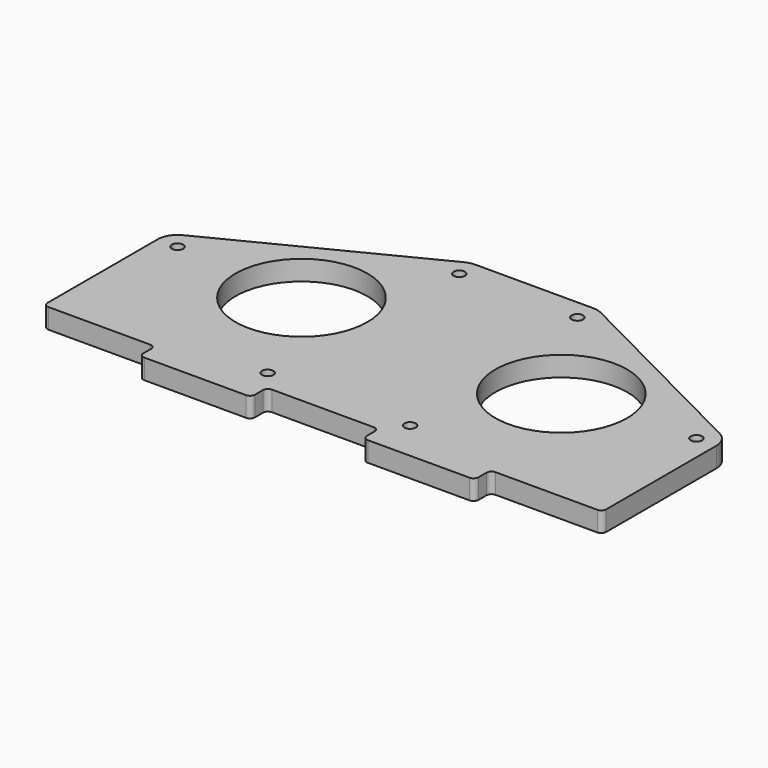
from build123d import *

# Parameters (mm, degrees)
F0_R     = 3.6195
F0_R_2   = 41.94175
F1_DEPTH = 12.7
F2_W     = 71.12
F2_H     = 12.7
F3_DEPTH = 12.7
F4_R     = 3.175


with BuildPart() as f1:
    # F0 (on Top) → F1 (new body)
    with BuildSketch(Plane.XY):
        with BuildLine():
            Line((37.5943482574, 0), (-37.5943482574, 0))
            ThreePointArc((-37.5943482574, 0), (-40.5487339943, -0.3484169064), (-43.3410161187, -1.3745504066))
            Line((-43.3410161187, -1.3745504066), (-170.8466678613, -66.0724350219))
            ThreePointArc((-170.8466678614, -66.0724350219), (-175.9229543527, -70.7530626401), (-177.8, -77.3978846153))
            Line((-177.8, -77.3978846153), (-177.8, -180.8720758428))
            Line((-177.8, -180.8720758428), (177.8, -180.8720758428))
            Line((177.8, -180.8720758428), (177.8, -77.3978846153))
            ThreePointArc((177.8, -77.3978846153), (175.9229543526, -70.7530626402), (170.8466678613, -66.0724350219))
            Line((170.8466678613, -66.0724350219), (43.3410161187, -1.3745504066))
            ThreePointArc((43.3410161187, -1.3745504066), (40.5487339943, -0.3484169064), (37.5943482574, 0))
        make_face()
        with Locations((-45.3171624807, -155.4720758428)):
            Circle(F0_R, mode=Mode.SUBTRACT)
        with Locations((45.3171624807, -155.4720758428)):
            Circle(F0_R, mode=Mode.SUBTRACT)
        with Locations((-165.1, -77.3978846153)):
            Circle(F0_R, mode=Mode.SUBTRACT)
        with Locations((-82.6705035794, -81.856653486)):
            Circle(F0_R_2, mode=Mode.SUBTRACT)
        with Locations((-37.5943482574, -12.7)):
            Circle(F0_R, mode=Mode.SUBTRACT)
        with Locations((82.6705035794, -81.856653486)):
            Circle(F0_R_2, mode=Mode.SUBTRACT)
        with Locations((165.1, -77.3978846153)):
            Circle(F0_R, mode=Mode.SUBTRACT)
        with Locations((37.5943482574, -12.7)):
            Circle(F0_R, mode=Mode.SUBTRACT)
    extrude(amount=F1_DEPTH)

    # F2 (on face) → F3 (cut, through all)
    with BuildSketch(Plane.XY.offset(12.7)):
        with Locations((-142.24, -174.5220758428)):
            Rectangle(F2_W, F2_H)
        with Locations((142.24, -174.5220758428)):
            Rectangle(F2_W, F2_H)
        with Locations((0, -174.5220758428)):
            Rectangle(F2_W, F2_H)
    extrude(amount=-F3_DEPTH, mode=Mode.SUBTRACT)

    # F4
    f4_edges = [f1.edges().sort_by_distance(p)[0] for p in [
        (-177.8, -168.172076, 6.35),
        (-106.68, -168.172076, 6.35),
        (-35.56, -168.172076, 6.35),
        (35.56, -168.172076, 6.35),
        (106.68, -168.172076, 6.35),
        (177.8, -168.172076, 6.35),
        (-106.68, -180.872076, 6.35),
        (-35.56, -180.872076, 6.35),
        (35.56, -180.872076, 6.35),
        (106.68, -180.872076, 6.35),
    ]]
    fillet(f4_edges, radius=F4_R)


solid = f1.part
